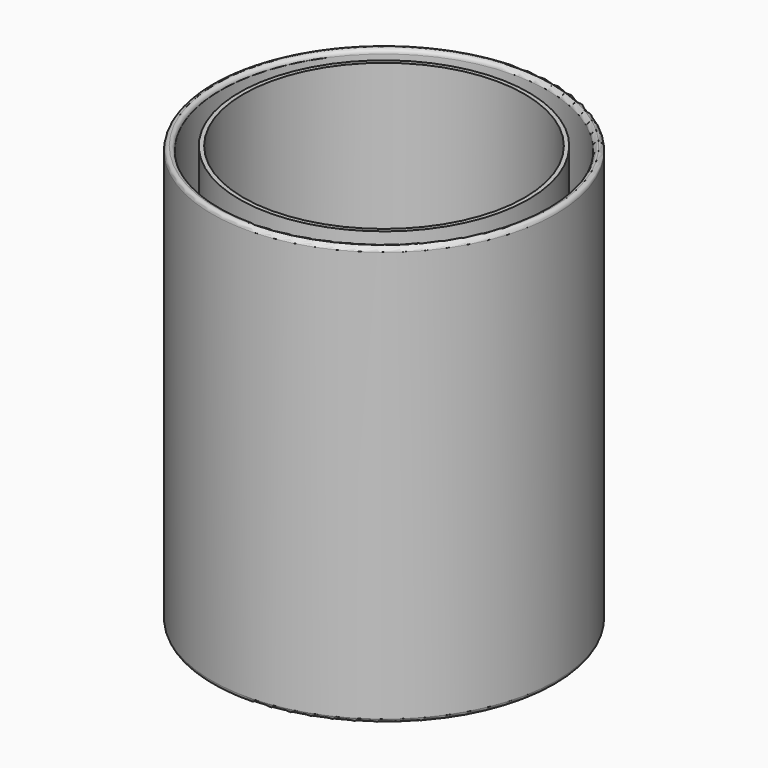
from build123d import *

# Parameters (mm, degrees)
F0_R     = 33.5
F1_DEPTH = 3
F2_R     = 34.5
F2_R_2   = 33.5
F3_DEPTH = 100
F4_R     = 41
F5_DEPTH = 3
F6_R     = 41
F6_R_2   = 39
F7_DEPTH = 100
F8_R     = 1
F9_R     = 0.99999


# Not quite as in the source:
# - a fillet or chamfer is up to 0.001 mm smaller than in the source, because OpenCascade refuses the exact size


with BuildPart() as f1:
    # F0 (on Top) → F1 (new body)
    with BuildSketch(Plane.XY):
        Circle(F0_R)
    extrude(amount=F1_DEPTH)

    # F2 (on Top) → F3 (join)
    with BuildSketch(Plane.XY):
        Circle(F2_R)
        Circle(F2_R_2, mode=Mode.SUBTRACT)
    extrude(amount=F3_DEPTH)

    # F4 (on Top) → F5 (join)
    with BuildSketch(Plane.XY):
        Circle(F4_R)
    extrude(amount=F5_DEPTH)

    # F6 (on Top) → F7 (join)
    with BuildSketch(Plane.XY):
        Circle(F6_R)
        Circle(F6_R_2, mode=Mode.SUBTRACT)
    extrude(amount=F7_DEPTH)

    # F8
    f8_edges = [f1.edges().sort_by_distance(p)[0] for p in [
        (-41, 0, 0),
    ]]
    fillet(f8_edges, radius=F8_R)

    # F9 (radius 1 in the source; OpenCascade refuses exactly that, so slightly less here)
    f9_edges = [f1.edges().sort_by_distance(p)[0] for p in [
        (-41, 0, 100),
        (-39, 0, 100),
    ]]
    fillet(f9_edges, radius=F9_R)


solid = f1.part
